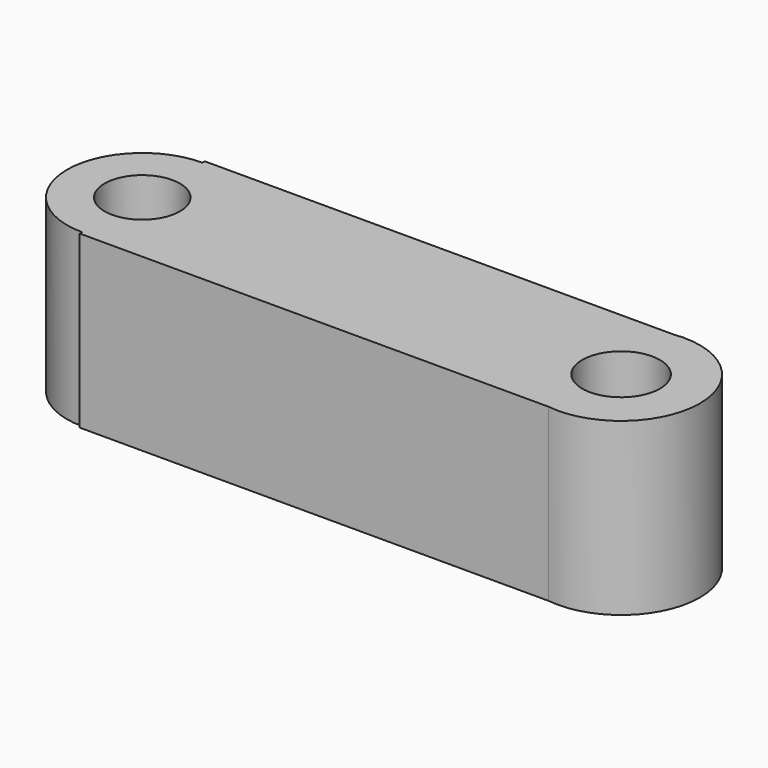
from build123d import *

# Parameters (mm, degrees)
F0_R     = 8.6737376807
F1_DEPTH = 25.4
F0_R_2   = 8.4076501903
F2_DEPTH = 38.1


# Not quite as in the source:
# - a feature names something its author has since deleted; it is built from what else it names


with BuildPart() as f1:
    # F0 (on Top) → F1 (new body)
    with BuildSketch(Plane.XY):
        with BuildLine():
            ThreePointArc((51.0823471633, -17.43234694), (70.9533001066, 0), (51.0823471633, 17.43234694))
            Line((51.0823471633, 17.43234694), (-53.3713176847, 17.43234694))
            Line((-53.3713176847, 17.43234694), (-53.3713176847, 16.7665737877))
            ThreePointArc((-53.3713176847, 16.7665737877), (-41.5155596621, 11.8557580225), (-36.604743897, 0))
            ThreePointArc((-36.604743897, 0), (-41.5155596621, -11.8557580225), (-53.3713176847, -16.7665737877))
            Line((-53.3713176847, -16.7665737877), (-53.3713176847, -17.43234694))
            Line((-53.3713176847, -17.43234694), (51.0823471633, -17.43234694))
        make_face()
        with Locations((53.3713176847, 0)):
            Circle(F0_R, mode=Mode.SUBTRACT)
    extrude(amount=F1_DEPTH)

    # F0 (on Top) → F2 (join)
    with BuildSketch(Plane.XY):
        with BuildLine():
            ThreePointArc((51.0823471633, -17.43234694), (70.9533001066, 0), (51.0823471633, 17.43234694))
            Line((51.0823471633, 17.43234694), (-53.3713176847, 17.43234694))
            Line((-53.3713176847, 17.43234694), (-53.3713176847, 16.7665737877))
            ThreePointArc((-53.3713176847, 16.7665737877), (-41.5155596621, 11.8557580225), (-36.604743897, 0))
            ThreePointArc((-36.604743897, 0), (-41.5155596621, -11.8557580225), (-53.3713176847, -16.7665737877))
            Line((-53.3713176847, -16.7665737877), (-53.3713176847, -17.43234694))
            Line((-53.3713176847, -17.43234694), (51.0823471633, -17.43234694))
        make_face()
        with Locations((53.3713176847, 0)):
            Circle(F0_R, mode=Mode.SUBTRACT)
        with BuildLine():
            ThreePointArc((-36.604743897, 0), (-41.5155596621, 11.8557580225), (-53.3713176847, 16.7665737877))
            ThreePointArc((-53.3713176847, 16.7665737877), (-70.1378914723, 0), (-53.3713176847, -16.7665737877))
            ThreePointArc((-53.3713176847, -16.7665737877), (-41.5155596621, -11.8557580225), (-36.604743897, 0))
        make_face()
        with Locations((-53.3713176847, 0)):
            Circle(F0_R_2, mode=Mode.SUBTRACT)
    extrude(amount=F2_DEPTH)


solid = f1.part
